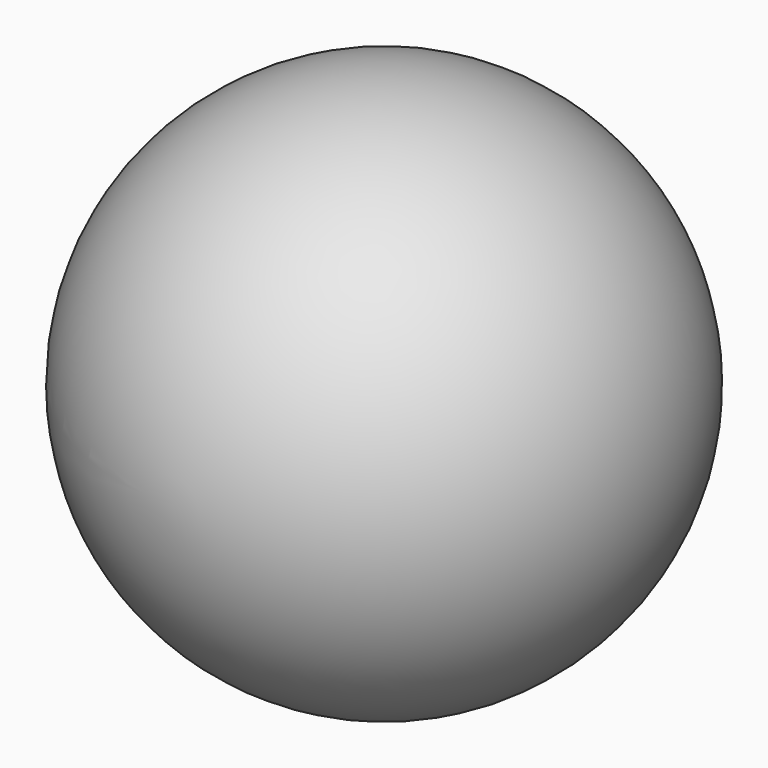
from build123d import *


with BuildPart() as f1:
    # F0 (on Top) → F1 (revolve)
    with BuildSketch(Plane.XY):
        with BuildLine():
            Line((0, -20.0025010854), (0, 52.6307395417))
            ThreePointArc((0, 52.6307395417), (-52.6307395417, 0), (0, -52.6307395417))
            Line((0, -52.6307395417), (0, -31.9123864174))
            add(Edge.make_bspline(
                [(0, -20.0025010854), (-3.9136368815, -19.8816393155), (-11.5859052169, -24.8774979415), (-4.0797572166, -31.6953563982), (0, -31.9123864174)],
                knots=[0.5059560827, 0.5059560827, 0.5059560827, 0.5059560827, 0.7471541801, 1, 1, 1, 1], degree=3))
        make_face()
        with BuildLine():
            add(Edge.make_bspline(
                [(-30.6908600032, 26.4155138284), (-30.4858879067, 26.9727110738), (-20.9428519895, 16.6649230466), (-5.3537528092, 32.6171085054), (-20.6467803964, 11.1687129283), (-30.9143408398, 25.808002325), (-30.6908600032, 26.4155138284)],
                knots=[0, 0, 0, 0, 0.2377537895, 0.481554644, 0.740777322, 1, 1, 1, 1], degree=3))
        make_face(mode=Mode.SUBTRACT)
        with BuildLine():
            Line((0, -31.9123864174), (0, -20.0025010854))
            add(Edge.make_bspline(
                [(0, -20.0025010854), (-3.9136368815, -19.8816393155), (-11.5859052169, -24.8774979415), (-4.0797572166, -31.6953563982), (0, -31.9123864174)],
                knots=[0.5059560827, 0.5059560827, 0.5059560827, 0.5059560827, 0.7471541801, 1, 1, 1, 1], degree=3))
        make_face()
    revolve(axis=Axis((0, -3.6883809259, 0), (0, -1, 0)))


solid = f1.part
